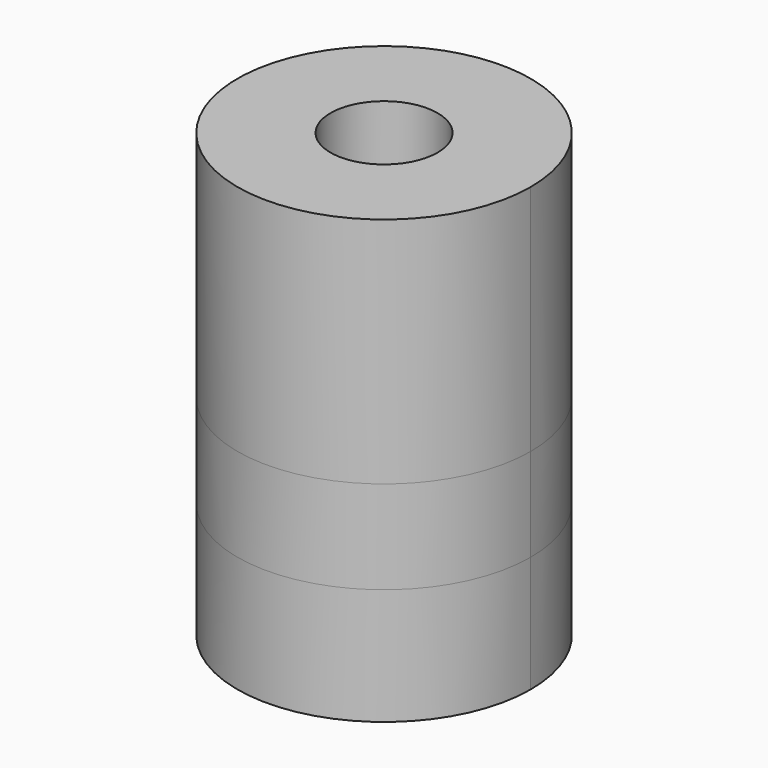
from build123d import *
from build123d import SkipClean  # not in build123d's __all__

# Parameters (mm, degrees)
F1_DEPTH = 4
F0_R     = 2.3
F2_DEPTH = 10
F3_DEPTH = 0.5
F4_DEPTH = 5


with BuildPart() as f1:
    # F0 (on Top) → F1 (new body)
    with BuildSketch(Plane.XY):
        with BuildLine():
            ThreePointArc((2.15, 4.6246621498), (4.2997092925, 2.7427176304), (5.1, 0))
            ThreePointArc((5.1, 0), (-2.7427176304, -4.2997092925), (-2.15, 4.6246621498))
            Line((-2.15, 4.6246621498), (-2.15, 5.9217818264))
            ThreePointArc((-2.15, 5.9217818264), (-3.615591238, -5.1592150566), (6.3, 0))
            ThreePointArc((6.3, 0), (5.1592150566, 3.615591238), (2.15, 5.9217818264))
            Line((2.15, 5.9217818264), (2.15, 4.6246621498))
        make_face()
    extrude(amount=-F1_DEPTH)

    # F0 (on Top) → F2 (join)
    with BuildSketch(Plane.XY):
        with BuildLine():
            ThreePointArc((2.15, 4.6246621498), (4.2997092925, 2.7427176304), (5.1, 0))
            ThreePointArc((5.1, 0), (-2.7427176304, -4.2997092925), (-2.15, 4.6246621498))
            Line((-2.15, 4.6246621498), (-2.15, 5.9217818264))
            ThreePointArc((-2.15, 5.9217818264), (-3.615591238, -5.1592150566), (6.3, 0))
            ThreePointArc((6.3, 0), (5.1592150566, 3.615591238), (2.15, 5.9217818264))
            Line((2.15, 5.9217818264), (2.15, 4.6246621498))
        make_face()
        with BuildLine():
            ThreePointArc((-2.15, 4.6246621498), (0, 5.1), (2.15, 4.6246621498))
            Line((2.15, 4.6246621498), (2.15, 5.9217818264))
            ThreePointArc((2.15, 5.9217818264), (0, 6.3), (-2.15, 5.9217818264))
            Line((-2.15, 5.9217818264), (-2.15, 4.6246621498))
        make_face()
        with BuildLine():
            ThreePointArc((-2.15, 4.6246621498), (-2.7427176304, -4.2997092925), (5.1, 0))
            ThreePointArc((5.1, 0), (4.2997092925, 2.7427176304), (2.15, 4.6246621498))
            Line((2.15, 4.6246621498), (-2.15, 4.6246621498))
        make_face()
        Circle(F0_R, mode=Mode.SUBTRACT)
        with BuildLine():
            Line((-2.15, 4.6246621498), (2.15, 4.6246621498))
            ThreePointArc((2.15, 4.6246621498), (0, 5.1), (-2.15, 4.6246621498))
        make_face()
    with SkipClean():  # cleaning this boolean's faces spoils the solid; the shape is the same uncleaned
        extrude(amount=F2_DEPTH)

    # F0 (on Top) → F3 (join)
    with BuildSketch(Plane.XY):
        with BuildLine():
            ThreePointArc((-2.15, 4.6246621498), (0, 5.1), (2.15, 4.6246621498))
            Line((2.15, 4.6246621498), (2.15, 5.9217818264))
            ThreePointArc((2.15, 5.9217818264), (0, 6.3), (-2.15, 5.9217818264))
            Line((-2.15, 5.9217818264), (-2.15, 4.6246621498))
        make_face()
    with SkipClean():  # cleaning this boolean's faces spoils the solid; the shape is the same uncleaned
        extrude(amount=-F3_DEPTH)

    # F4 (add): a face of the model
    f4_faces = [f1.faces().sort_by_distance(p)[0] for p in [
        (2.3255368768, 5.2732219881, -4),
    ]]
    with SkipClean():  # cleaning this boolean's faces spoils the solid; the shape is the same uncleaned
        extrude(f4_faces, amount=F4_DEPTH)


solid = f1.part
